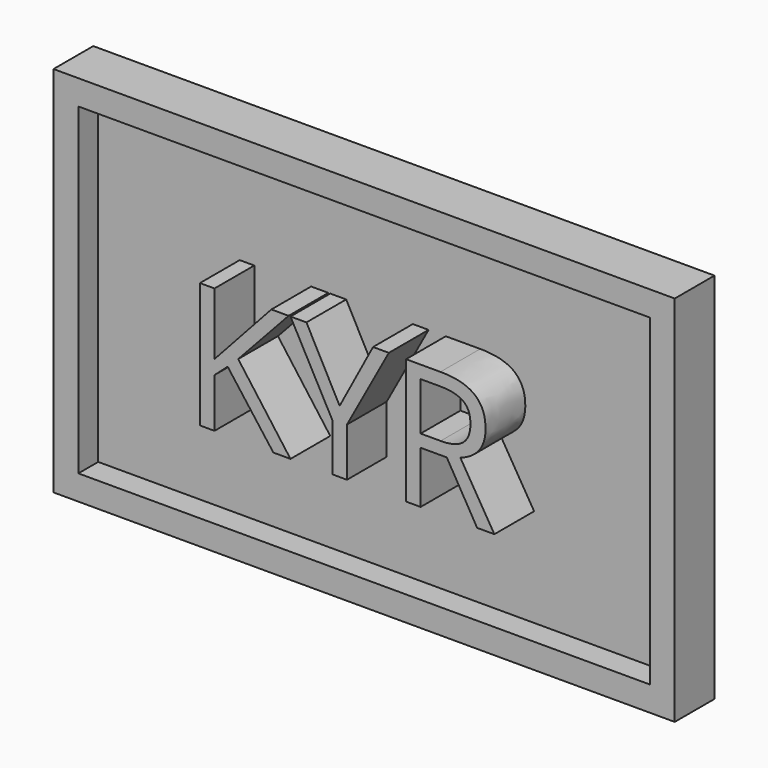
from build123d import *

# Parameters (mm, degrees)
F0_W         = 250
F0_H         = 150
F1_DEPTH     = 20
F2_W         = 230
F2_H         = 130
F3_DEPTH     = 10
F4_W         = 160
F4_H         = 80
F5_DEPTH     = 10
F6_R         = 14
F7_DEPTH     = 25
F8_TEXT_SIZE = 70.6641753015
F9_DEPTH     = 20


# Not quite as in the source:
# - Text() gives the source's letters only with a copy of the font that has no kerning and outlines rounded to 1/6400 em; it was checked with that copy


with BuildPart() as f1:
    # F0 (on Front) → F1 (new body)
    with BuildSketch(Plane.XZ):
        Rectangle(F0_W, F0_H)
    extrude(amount=F1_DEPTH)

    # F2 (on face) → F3 (cut)
    with BuildSketch(Plane.XZ.offset(20)):
        Rectangle(F2_W, F2_H)
    extrude(amount=-F3_DEPTH, mode=Mode.SUBTRACT)

    # F4 (on face) → F5 (join)
    with BuildSketch(Plane(origin=(0, 0, 0), x_dir=(-1, 0, 0), z_dir=(0, 1, 0))):
        Rectangle(F4_W, F4_H)
    extrude(amount=F5_DEPTH)

    # F6 (on face) → F7 (join)
    with BuildSketch(Plane(origin=(0, 10, 0), x_dir=(-1, 0, 0), z_dir=(0, 1, 0))):
        Circle(F6_R)
    extrude(amount=F7_DEPTH)

    # F8 (on face) → F9 (join)
    with BuildSketch(Plane.XZ.offset(10)):
        with Locations((-65, -25.4391031085)):
            Text('KYR', F8_TEXT_SIZE, font='Open Sans', text_align=(TextAlign.LEFT, TextAlign.BOTTOM))
    extrude(amount=F9_DEPTH)


solid = f1.part
